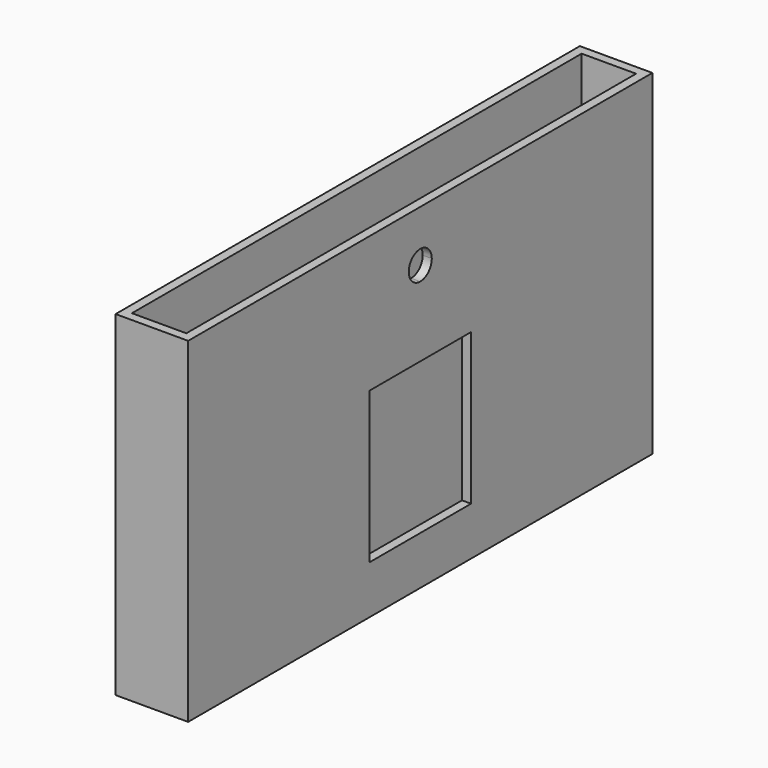
from build123d import *

# Parameters (mm, degrees)
F0_W     = 152.4
F0_H     = 1219.2
F0_W_2   = 114.3
F0_H_2   = 1181.1
F1_DEPTH = 704.85
F3_DEPTH = 25.4
F5_DEPTH = 25.4


# Not quite as in the source:
# - a feature names something its author has since deleted; it is built from what else it names


with BuildPart() as f1:
    # F0 (on Top) → F1 (new body)
    with BuildSketch(Plane.XY):
        Rectangle(F0_W, F0_H)
        Rectangle(F0_W_2, F0_H_2, mode=Mode.SUBTRACT)
    extrude(amount=F1_DEPTH)

    # F2 (on face) → F3 (cut)
    with BuildSketch(Plane.YZ.offset(76.2)):
        with BuildLine():
            ThreePointArc((30.226, 596.9), (-21.3730095681, 618.2730095681), (0, 566.674))
            ThreePointArc((0, 566.674), (21.3730095681, 575.5269904319), (30.226, 596.9))
        make_face()
        Polygon((-133.35, 101.6), (0, 101.6), (133.35, 101.6), (133.35, 419.1), (0, 419.1), (-133.35, 419.1), align=None)
    extrude(amount=-F3_DEPTH, mode=Mode.SUBTRACT)

    # F4 (on face) → F5 (cut)
    with BuildSketch(Plane(origin=(-76.2, 0, 0), x_dir=(0, -1, 0), z_dir=(-1, 0, 0))):
        with BuildLine():
            ThreePointArc((30.226, 406.4), (-21.3730095681, 427.7730095681), (0, 376.174))
            ThreePointArc((0, 376.174), (21.3730095681, 385.0269904319), (30.226, 406.4))
        make_face()
    extrude(amount=-F5_DEPTH, mode=Mode.SUBTRACT)


solid = f1.part
